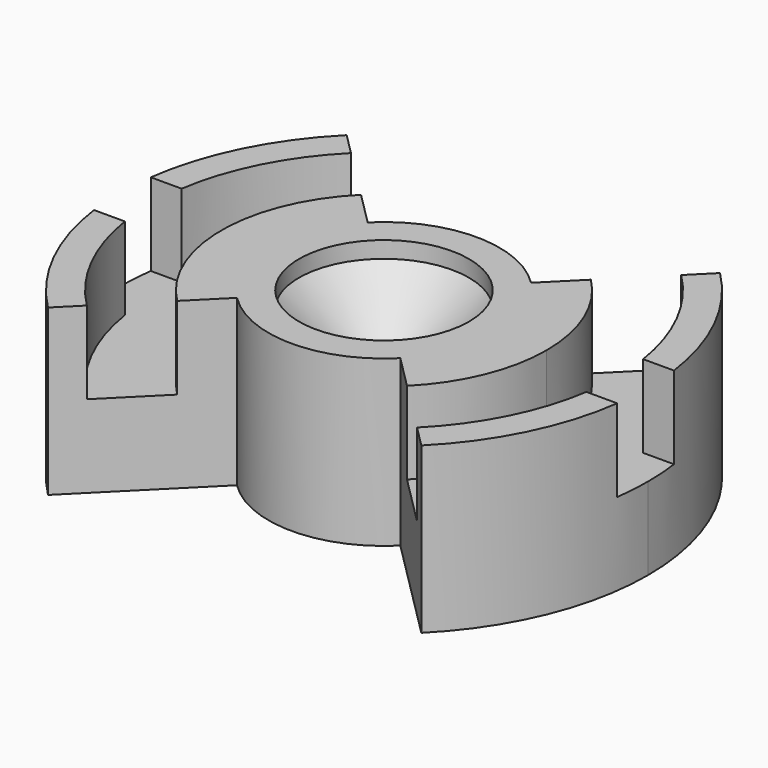
from build123d import *

# Parameters (mm, degrees)
F0_R     = 3.27025
F1_DEPTH = 6.35
F2_R     = 3.27025
F3_DEPTH = 3.175
F4_SIZE  = 2.54


# Not quite as in the source:
# - a feature names something its author has since deleted; it is built from what else it names


with BuildPart() as f1:
    # F0 (on Top) → F1 (new body)
    with BuildSketch(Plane.XY):
        with BuildLine():
            ThreePointArc((-4.445, 0), (-4.106644522, 1.7010278569), (-3.1430896424, 3.1430896424))
            Line((-3.1430896424, 3.1430896424), (-7.1842048969, 7.1842048969))
            ThreePointArc((-7.1842048969, 7.1842048969), (-9.3866160503, 3.8880636728), (-10.16, 0))
            ThreePointArc((-10.16, 0), (-9.3866160503, -3.8880636728), (-7.1842048969, -7.1842048969))
            Line((-7.1842048969, -7.1842048969), (-3.1430896424, -3.1430896424))
            ThreePointArc((-3.1430896424, -3.1430896424), (-4.106644522, -1.7010278569), (-4.445, 0))
        make_face()
        with BuildLine():
            ThreePointArc((3.1430896424, -3.1430896424), (4.106644522, -1.7010278569), (4.445, 0))
            ThreePointArc((4.445, 0), (4.106644522, 1.7010278569), (3.1430896424, 3.1430896424))
            ThreePointArc((3.1430896424, 3.1430896424), (0, 4.445), (-3.1430896424, 3.1430896424))
            ThreePointArc((-3.1430896424, 3.1430896424), (-4.106644522, 1.7010278569), (-4.445, 0))
            ThreePointArc((-4.445, 0), (-4.106644522, -1.7010278569), (-3.1430896424, -3.1430896424))
            ThreePointArc((-3.1430896424, -3.1430896424), (0, -4.445), (3.1430896424, -3.1430896424))
        make_face()
        Circle(F0_R, mode=Mode.SUBTRACT)
        with BuildLine():
            ThreePointArc((3.1430896424, 3.1430896424), (4.106644522, 1.7010278569), (4.445, 0))
            ThreePointArc((4.445, 0), (4.106644522, -1.7010278569), (3.1430896424, -3.1430896424))
            Line((3.1430896424, -3.1430896424), (7.1842048969, -7.1842048969))
            ThreePointArc((7.1842048969, -7.1842048969), (9.3866160503, -3.8880636728), (10.16, 0))
            ThreePointArc((10.16, 0), (9.3866160503, 3.8880636728), (7.1842048969, 7.1842048969))
            Line((7.1842048969, 7.1842048969), (3.1430896424, 3.1430896424))
        make_face()
        Circle(F0_R)
    extrude(amount=F1_DEPTH)

    # F2 (on face) → F3 (cut)
    with BuildSketch(Plane.XY.offset(6.35)):
        with BuildLine():
            ThreePointArc((-4.4227761396, -4.4227761396), (-6.25475, 0), (-4.4227761396, 4.4227761396))
            Line((-4.4227761396, 4.4227761396), (-6.3535312057, 6.3535312057))
            ThreePointArc((-6.3535312057, 6.3535312057), (-8.0151664506, 4.0610127224), (-8.8809239384, 1.36525))
            ThreePointArc((-8.8809239384, 1.36525), (-8.98525, 0), (-8.8809239384, -1.36525))
            ThreePointArc((-8.8809239384, -1.36525), (-8.0151664506, -4.0610127224), (-6.3535312057, -6.3535312057))
            Line((-6.3535312057, -6.3535312057), (-4.4227761396, -4.4227761396))
        make_face()
        with BuildLine():
            ThreePointArc((4.4227761396, 4.4227761396), (5.778635506, 2.3935891986), (6.25475, 0))
            ThreePointArc((6.25475, 0), (5.778635506, -2.3935891986), (4.4227761396, -4.4227761396))
            Line((4.4227761396, -4.4227761396), (6.3535312057, -6.3535312057))
            ThreePointArc((6.3535312057, -6.3535312057), (8.0151664506, -4.0610127224), (8.8809239384, -1.36525))
            ThreePointArc((8.8809239384, -1.36525), (8.9591305209, -0.6846151272), (8.98525, 0))
            ThreePointArc((8.98525, 0), (8.9591305209, 0.6846151272), (8.8809239384, 1.36525))
            ThreePointArc((8.8809239384, 1.36525), (8.0151664506, 4.0610127224), (6.3535312057, 6.3535312057))
            Line((6.3535312057, 6.3535312057), (4.4227761396, 4.4227761396))
        make_face()
        with BuildLine():
            ThreePointArc((-8.8809239384, -1.36525), (-8.98525, 0), (-8.8809239384, 1.36525))
            Line((-8.8809239384, 1.36525), (-10.0678544108, 1.36525))
            ThreePointArc((-10.0678544108, 1.36525), (-10.16, 0), (-10.0678544108, -1.36525))
            Line((-10.0678544108, -1.36525), (-8.8809239384, -1.36525))
        make_face()
        with BuildLine():
            Line((10.0678544108, 1.36525), (8.8809239384, 1.36525))
            ThreePointArc((8.8809239384, 1.36525), (8.9591305209, 0.6846151272), (8.98525, 0))
            ThreePointArc((8.98525, 0), (8.9591305209, -0.6846151272), (8.8809239384, -1.36525))
            Line((8.8809239384, -1.36525), (10.0678544108, -1.36525))
            ThreePointArc((10.0678544108, -1.36525), (10.16, 0), (10.0678544108, 1.36525))
        make_face()
        Circle(F2_R)
    extrude(amount=-F3_DEPTH, mode=Mode.SUBTRACT)

    # F4
    f4_edges = [f1.edges().sort_by_distance(p)[0] for p in [
        (-3.27025, 0, 3.175),
    ]]
    chamfer(f4_edges, length=F4_SIZE)


solid = f1.part
